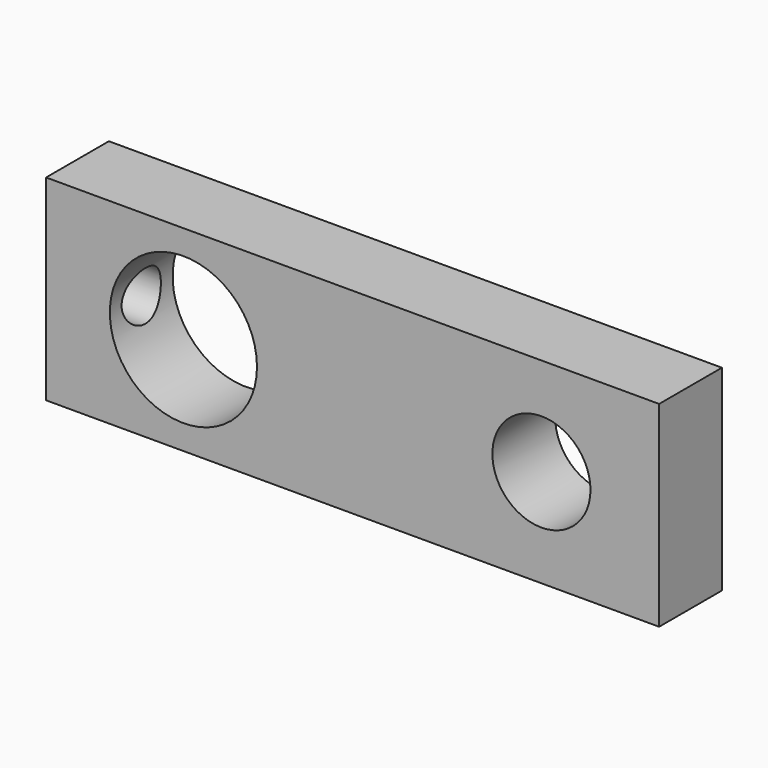
from build123d import *

# Parameters (mm, degrees)
F0_W     = 62.5
F0_H     = 20
F0_R     = 7.5
F0_R_2   = 5
F1_DEPTH = 5.5
F2_DEPTH = 2.5
F3_R     = 2.5
F4_DEPTH = 10


# Not quite as in the source:
# - a feature names something its author has since deleted; it is built from what else it names


with BuildPart() as f1:
    # F0 (on Front) → F1 (new body)
    with BuildSketch(Plane.XZ):
        with Locations((-2, 0)):
            Rectangle(F0_W, F0_H)
        with Locations((-19.25, 0)):
            Circle(F0_R, mode=Mode.SUBTRACT)
        with Locations((17.25, 0)):
            Circle(F0_R_2, mode=Mode.SUBTRACT)
    extrude(amount=F1_DEPTH)

    # F2 (add): a face of the model
    f2_faces = [f1.faces().sort_by_distance(p)[0] for p in [
        (-0.4554491501, -5.5, 0),
    ]]
    extrude(f2_faces, amount=F2_DEPTH)

    # F3 (on face) → F4 (cut)
    with BuildSketch(Plane(origin=(-33.25, 0, 0), x_dir=(0, -1, 0), z_dir=(-1, 0, 0))):
        with Locations((4, 0)):
            Circle(F3_R)
    extrude(amount=-F4_DEPTH, mode=Mode.SUBTRACT)


solid = f1.part
